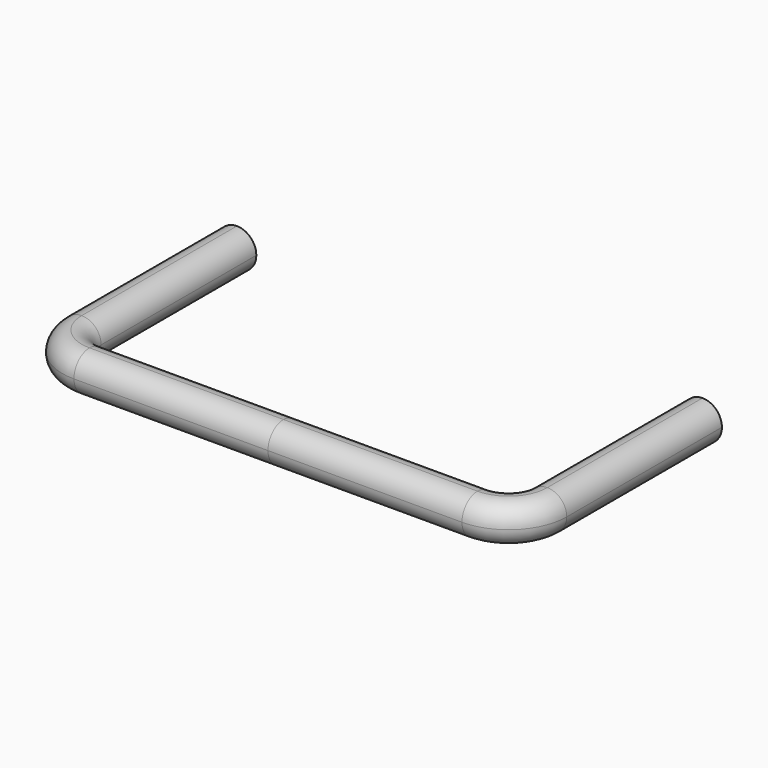
from build123d import *

# Parameters (mm, degrees)
F1_DEPTH = 5
F2_R     = 4.99999


# Not quite as in the source:
# - a fillet or chamfer is up to 0.001 mm smaller than in the source, because OpenCascade refuses the exact size
# - ends of sketch curves that miss each other by under 0.0002 mm in the source are joined


with BuildPart() as f1:
    # F0 (on Top) → F1 (new body, symmetric)
    with BuildSketch(Plane.XY):
        with BuildLine():
            Line((-55, 42.9439264748), (-65, 42.9439264748))
            Line((-65, 42.9439264748), (-65, -7.0560735252))
            ThreePointArc((-65, -7.0560735252), (-60.6066017178, -17.662675243), (-50, -22.0560735252))
            Line((-50, -22.0560735252), (0, -22.0560735252))
            Line((0, -22.0560735252), (50, -22.0560729504))
            ThreePointArc((50, -22.0560729504), (60.6066017178, -17.662675243), (65, -7.0560735252))
            Line((65, -7.0560735252), (65.000000149, 42.9439264748))
            Line((65.000000149, 42.9439264748), (55, 42.9439264748))
            Line((55, 42.9439264748), (55, -7.0560735252))
            ThreePointArc((55, -7.0560735252), (53.5355343776, -10.5916079028), (50, -12.0560741922))
            Line((50, -12.0560741922), (0, -12.0560735252))
            Line((0, -12.0560735252), (-50, -12.0560735252))
            ThreePointArc((-50, -12.0560735252), (-53.5355343776, -10.5916079028), (-55.000000667, -7.0560735252))
            Line((-55.000000667, -7.0560735252), (-55, 42.9439264748))
        make_face()
    extrude(amount=F1_DEPTH, both=True)

    # F2 (radius 5 in the source; OpenCascade refuses exactly that, so slightly less here)
    f2_edges = [f1.edges().sort_by_distance(p)[0] for p in [
        (-65, 17.943926, 5),
        (-65, -7.056074, 0),
        (-60.606602, -17.662675, -5),
        (-50, -22.056074, 0),
        (-60.606602, -17.662675, 5),
        (-25, -22.056074, -5),
        (0, -22.056074, 0),
        (-25, -22.056074, 5),
        (50, -22.056073, 0),
        (60.606602, -17.662675, -5),
        (65, -7.056074, 0),
        (60.606602, -17.662675, 5),
        (55, -7.056074, 0),
        (53.535534, -10.591608, -5),
        (50, -12.056074, 0),
        (53.535534, -10.591608, 5),
        (-25, -12.056074, -5),
        (-50, -12.056074, 0),
        (-25, -12.056074, 5),
        (0, -12.056074, 0),
        (-53.535534, -10.591608, -5),
        (-55.000001, -7.056074, 0),
        (-53.535534, -10.591608, 5),
    ]]
    fillet(f2_edges, radius=F2_R)


solid = f1.part
